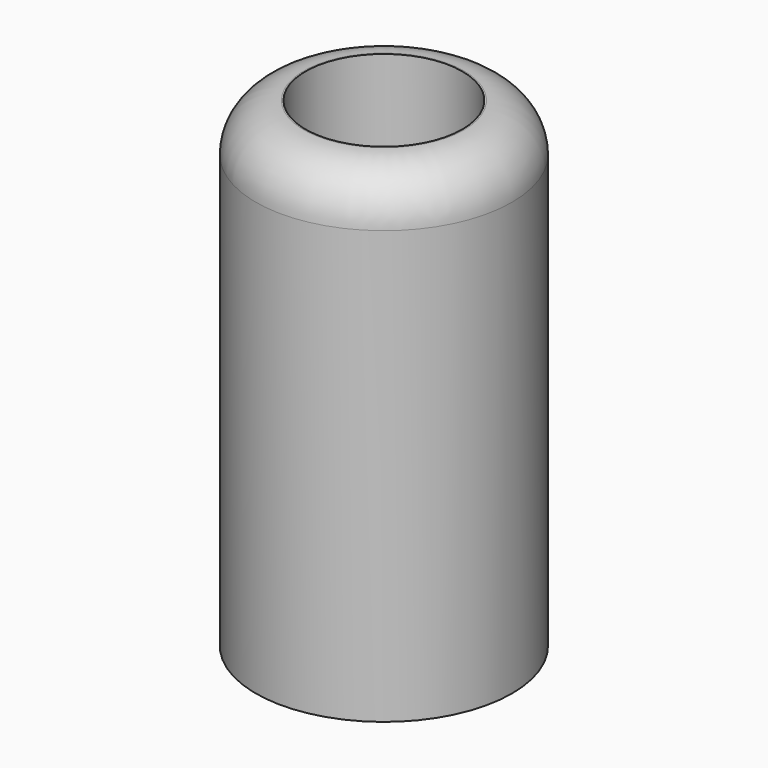
from build123d import *

# Parameters (mm, degrees)
F0_R         = 8
F1_DEPTH     = 30
F3_R         = 4.9
F4_DEPTH     = 22.3
F6_TEXT_SIZE = 8.7760906253
F7_DEPTH     = 3
F8_R         = 3


# Not quite as in the source:
# - Text() gives the source's letters only with a copy of the font that has no kerning and outlines rounded to 1/6400 em; it was checked with that copy


with BuildPart() as f1:
    # F0 (on Top) → F1 (new body)
    with BuildSketch(Plane.XY):
        Circle(F0_R)
    extrude(amount=F1_DEPTH)

    # F3 (on offset) → F4 (cut)
    with BuildSketch(Plane.XY.offset(30)):
        Circle(F3_R)
    extrude(amount=-F4_DEPTH, mode=Mode.SUBTRACT)

    # F6 (on offset) → F7 (cut)
    with BuildSketch(Plane(origin=(0, 0, 0), x_dir=(1, 0, 0), z_dir=(0, 0, -1))):
        with Locations((-6.4837737009, -3.2532070763)):
            Text('3/8', F6_TEXT_SIZE, font='Open Sans', font_style=FontStyle.BOLD, text_align=(TextAlign.LEFT, TextAlign.BOTTOM))
    extrude(amount=-F7_DEPTH, mode=Mode.SUBTRACT)

    # F8
    f8_edges = [f1.edges().sort_by_distance(p)[0] for p in [
        (-8, 0, 30),
    ]]
    fillet(f8_edges, radius=F8_R)


solid = f1.part
